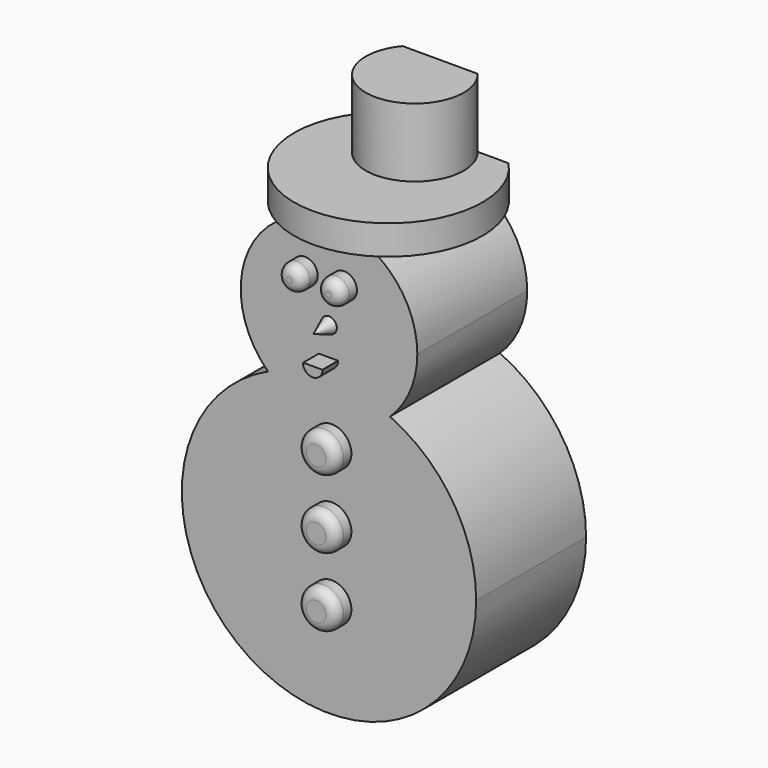
from build123d import *

# Parameters (mm, degrees)
F1_DEPTH  = 7
F2_DEPTH  = 7
F3_R      = 1
F4_DEPTH  = 1
F5_DEPTH  = 1
F6_DEPTH  = 1
F7_R      = 0.65
F8_DEPTH  = 1
F9_DEPTH  = 1
F14_DEPTH = 1.5
F16_DEPTH = 3.5
F18_DEPTH = 1
F19_R     = 0.5


# Not quite as in the source:
# - a feature names something its author has since deleted; it is built from what else it names


with BuildPart() as f1:
    # F0 (on Front) → F1 (new body)
    with BuildSketch(Plane.XZ):
        with BuildLine():
            ThreePointArc((-3.1083265336, 6.8255626992), (0, 5.5795304558), (3.1083265336, 6.8255626992))
            ThreePointArc((3.1083265336, 6.8255626992), (0, 7.5), (-3.1083265336, 6.8255626992))
        make_face()
        with BuildLine():
            ThreePointArc((-3.1083265336, 6.8255626992), (0, 7.5), (3.1083265336, 6.8255626992))
            ThreePointArc((3.1083265336, 6.8255626992), (4.1374792689, 8.3099922958), (4.5, 10.0795304558))
            ThreePointArc((4.5, 10.0795304558), (-1.7695381599, 14.2170097247), (-3.1083265336, 6.8255626992))
        make_face()
    extrude(amount=F1_DEPTH)

    # F0 (on Front) → F2 (join)
    with BuildSketch(Plane.XZ):
        with BuildLine():
            ThreePointArc((-3.1083265336, 6.8255626992), (-4.0581739119, -6.3072358844), (7.5, 0))
            ThreePointArc((7.5, 0), (6.3072358844, 4.0581739119), (3.1083265336, 6.8255626992))
            ThreePointArc((3.1083265336, 6.8255626992), (0, 5.5795304558), (-3.1083265336, 6.8255626992))
        make_face()
    extrude(amount=F2_DEPTH)

    # F3 (on face) → F4 (join)
    with BuildSketch(Plane.XZ.offset(7)):
        with Locations((0.1404315871, 4.5206134686)):
            Circle(F3_R)
    extrude(amount=F4_DEPTH)

    # F3 (on face) → F5 (join)
    with BuildSketch(Plane.XZ.offset(7)):
        with Locations((0.1404315871, 1.0206134686)):
            Circle(F3_R)
    extrude(amount=F5_DEPTH)

    # F3 (on face) → F6 (join)
    with BuildSketch(Plane.XZ.offset(7)):
        with Locations((0.1404315871, -2.4793865314)):
            Circle(F3_R)
    extrude(amount=F6_DEPTH)

    # F7 (on face) → F8 (join)
    with BuildSketch(Plane.XZ.offset(7)):
        with Locations((-1.2232928476, 11.9385918571)):
            Circle(F7_R)
    extrude(amount=F8_DEPTH)

    # F7 (on face) → F9 (join)
    with BuildSketch(Plane.XZ.offset(7)):
        with Locations((0.7767071524, 11.9385918571)):
            Circle(F7_R)
    extrude(amount=F9_DEPTH)

    # F10 (on Right) → F11 (revolve)
    with BuildSketch(Plane.YZ):
        Polygon((-7.9928543597, 9.9160444998), (-6.9928543597, 9.9160444998), (-6.9928543597, 10.3160444998), align=None)
    revolve(axis=Axis((0, -7.4928543597, 9.9160444998), (0, -1, 0)))

    # F13 (on offset) → F14 (join)
    with BuildSketch(Plane.XY.offset(14)):
        with BuildLine():
            Line((3.561746113, -0.0150235719), (-3.438253887, -0.0150235719))
            ThreePointArc((-3.438253887, -0.0150235719), (0.061746113, -8.099837113), (3.561746113, -0.0150235719))
        make_face()
    extrude(amount=F14_DEPTH)

    # F15 (on face) → F16 (join)
    with BuildSketch(Plane.XY.offset(15.5)):
        with BuildLine():
            Line((1.9837659688, -0.0150235719), (-1.8346020611, -0.0150235719))
            ThreePointArc((-1.8346020611, -0.0150235719), (0.0745819538, -4.1290298907), (1.9837659688, -0.0150235719))
        make_face()
    extrude(amount=F16_DEPTH)

    # F17 (on face) → F18 (join)
    with BuildSketch(Plane.XZ.offset(7)):
        with BuildLine():
            Line((0.4505876301, 8.4716784917), (-0.5113184951, 8.4716784917))
            ThreePointArc((-0.5113184951, 8.4716784917), (-0.5247841756, 8.4659470606), (-0.5299885637, 8.4522690419))
            ThreePointArc((-0.5299885637, 8.4522690419), (-0.0303654325, 7.9716784917), (0.4692576987, 8.4522690419))
            ThreePointArc((0.4692576987, 8.4522690419), (0.4640533106, 8.4659470606), (0.4505876301, 8.4716784917))
        make_face()
    extrude(amount=F18_DEPTH)

    # F19
    f19_edges = [f1.edges().sort_by_distance(p)[0] for p in [
        (-1.873293, -8, 11.938592),
        (0.126707, -8, 11.938592),
        (-0.859568, -8, 4.520613),
        (-0.859568, -8, 1.020613),
        (-0.859568, -8, -2.479387),
    ]]
    fillet(f19_edges, radius=F19_R)


solid = f1.part
